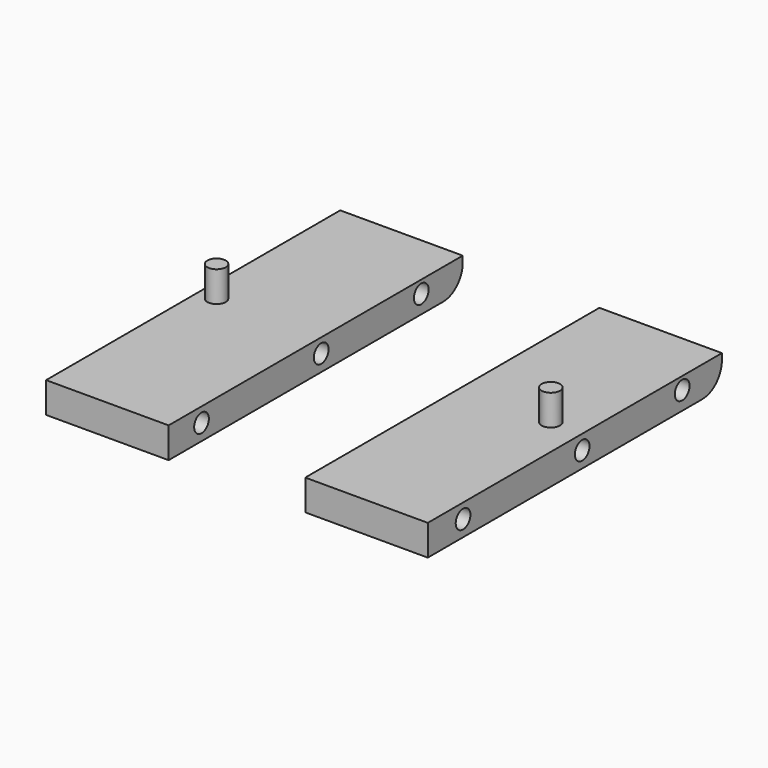
from build123d import *

# Parameters (mm, degrees)
F0_W     = 25.4
F0_H     = 76.2
F1_DEPTH = 6.35
F2_R     = 5.08
F2_2_R   = 5.08
F3_R     = 1.905
F4_DEPTH = 127
F6_R     = 1.905
F7_DEPTH = 6.35
F5_R     = 1.905
F8_DEPTH = 101.6


with BuildPart() as f1:
    # F0 (on Top) → F1 (new body)
    with BuildSketch(Plane.XY):
        with Locations((-32.0039651388, -1.4284911171)):
            Rectangle(F0_W, F0_H)
    extrude(amount=F1_DEPTH)

    # F2
    f2_edges = [f1.edges().sort_by_distance(p)[0] for p in [
        (-32.003965, 36.671509, 0),
    ]]
    fillet(f2_edges, radius=F2_R)

    # F3 (on face) → F4 (cut)
    with BuildSketch(Plane(origin=(-44.7039651388, 0, 0), x_dir=(0, -1, 0), z_dir=(-1, 0, 0))):
        with Locations((-25.9214825928, 3.745357506)):
            Circle(F3_R)
        with Locations((0, 3.3983075991)):
            Circle(F3_R)
        with Locations((31.0074724257, 3.3381541725)):
            Circle(F3_R)
    extrude(amount=-F4_DEPTH, mode=Mode.SUBTRACT)


with BuildPart() as f1b:
    # F0 (on Top) → F1, piece 2 (new body)
    with BuildSketch(Plane.XY):
        with Locations((22.0886249452, -1.8988993988)):
            Rectangle(F0_W, F0_H)
    extrude(amount=F1_DEPTH)

    # F2#2
    f2_2_edges = [f1b.edges().sort_by_distance(p)[0] for p in [
        (22.088625, 36.201101, 0),
    ]]
    fillet(f2_2_edges, radius=F2_2_R)

    # F5 (on face) → F8 (cut)
    with BuildSketch(Plane(origin=(9.3886249452, 0, 0), x_dir=(0, -1, 0), z_dir=(-1, 0, 0))):
        with Locations((-25.9032901376, 3.7854171824)):
            Circle(F5_R)
        with Locations((0, 3.3236292657)):
            Circle(F5_R)
        with Locations((30.860632658, 3.3236292657)):
            Circle(F5_R)
    extrude(amount=-F8_DEPTH, mode=Mode.SUBTRACT)


with BuildPart() as f7:
    # F6 (on face) → F7 (new body)
    with BuildSketch(Plane.XY.offset(6.35)):
        with Locations((-40.9925282001, 0)):
            Circle(F6_R)
    extrude(amount=F7_DEPTH)


with BuildPart() as f7b:
    # F6 (on face) → F7, piece 2 (new body)
    with BuildSketch(Plane.XY.offset(6.35)):
        with Locations((28.2885536096, 0)):
            Circle(F6_R)
    extrude(amount=F7_DEPTH)


solid = Compound([f1.part, f1b.part, f7.part, f7b.part])
